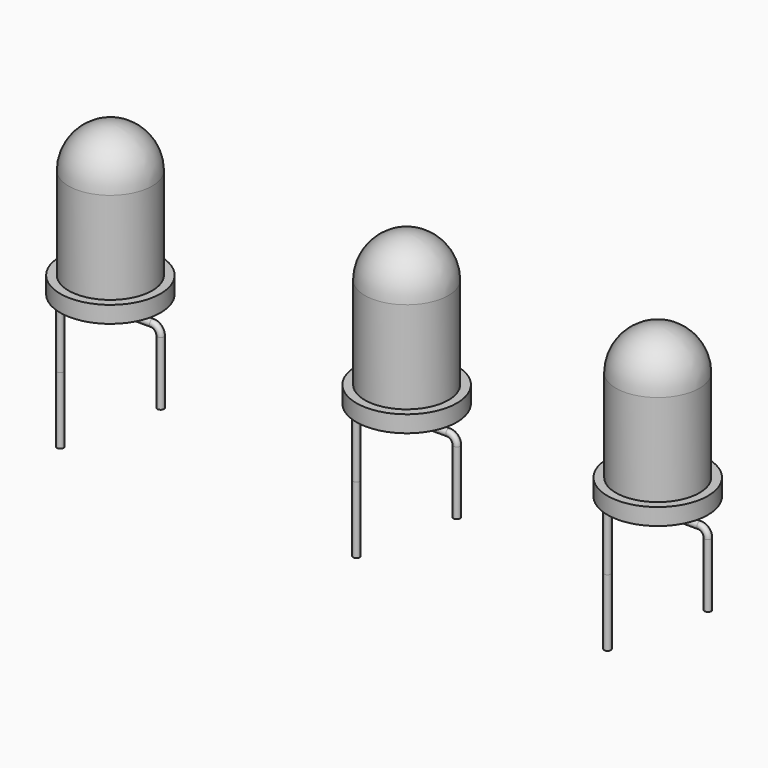
from build123d import *

# Parameters (mm, degrees)
F3_R     = 0.2
F5_R     = 0.2
F6_DEPTH = 4


# Not quite as in the source:
# - a pattern or mirror of a feature is missing from the dataset's text; its kind, count and spacing are read off the source's solid


with BuildPart() as f1:
    # F0 (on Front) → F1 (revolve)
    with BuildSketch(Plane.XZ):
        with BuildLine():
            Line((2.5, 1), (2.5, 6.5))
            ThreePointArc((2.5, 6.5), (1.767766953, 4.732233047), (0, 4))
            Line((0, 4), (0, 0))
            Line((0, 0), (3, 0))
            Line((3, 0), (3, 1))
            Line((3, 1), (2.5, 1))
        make_face()
        with BuildLine():
            ThreePointArc((0, 4), (1.767766953, 4.732233047), (2.5, 6.5))
            ThreePointArc((2.5, 6.5), (1.767766953, 8.267766953), (0, 9))
            Line((0, 9), (0, 6.5))
            Line((0, 6.5), (0, 4))
        make_face()
    revolve(axis=Axis((0, 0, 3.25), (0, 0, -1)))

    # F4: sweep along a path in F2
    with BuildLine(Plane.XZ) as f4_path:
        Line((1.2, 0), (1.2, -0.2))
        ThreePointArc((1.2, -0.2), (1.3464466094, -0.5535533906), (1.7, -0.7))
        Line((1.7, -0.7), (2.5, -0.7))
        ThreePointArc((2.5, -0.7), (2.8535533906, -0.8464466094), (3, -1.2))
        Line((3, -1.2), (3, -5))
    # F3 (on Top) → F4 (sweep)
    with BuildSketch(Plane.XY):
        with Locations((1.2, 0)):
            Circle(F3_R)
    f4 = sweep(path=f4_path.line)

    # F4_copies: F4 across plane
    add(f4.mirror(Plane(origin=(0, 0, 0), x_dir=(0, 0, -1), z_dir=(-1, 0, 0))))

    # F5 (on face) → F6 (join)
    with BuildSketch(Plane(origin=(0, 0, -5), x_dir=(1, 0, 0), z_dir=(0, 0, -1))):
        with Locations((-3, 0)):
            Circle(F5_R)
    extrude(amount=F6_DEPTH)


with BuildPart() as f7_1:
    # F7: copy of F1
    add(f1.part.moved(Location((17.7, 0, 0))))


with BuildPart() as f8_1:
    # F8: copy of F1
    add(f1.part.moved(Location((32.7, 0, 0))))


solid = Compound([f1.part, f7_1.part, f8_1.part])
